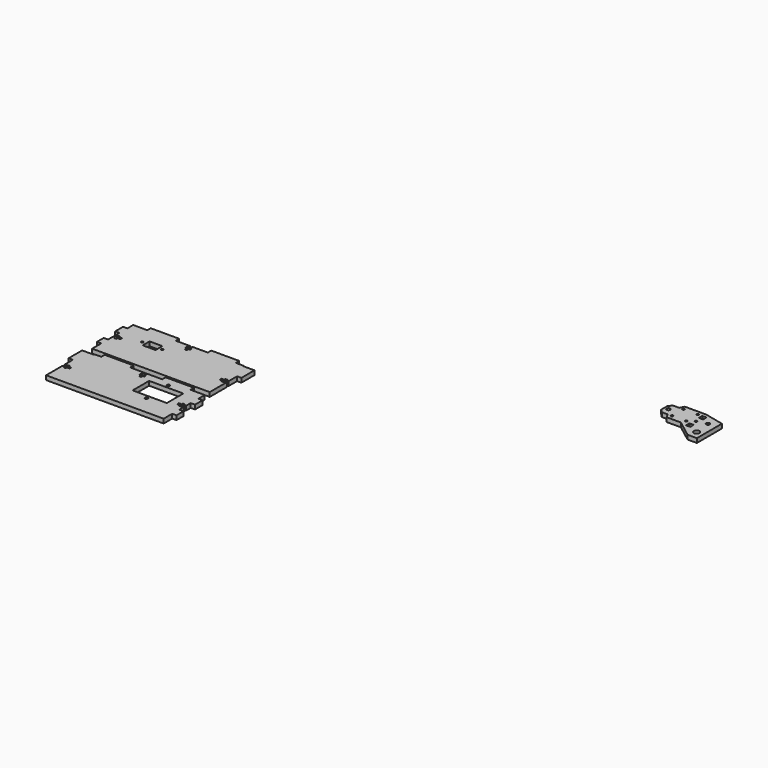
from build123d import *

# Parameters (mm, degrees)
F0_R     = 2
F0_W     = 48
F0_H     = 29
F1_DEPTH = 6
F0_R_2   = 1.5
F0_W_2   = 18
F0_H_2   = 12
F2_DEPTH = 6
F0_R_3   = 4
F0_W_3   = 6
F0_H_3   = 6
F0_R_4   = 2.5
F3_DEPTH = 6


# Not quite as in the source:
# - a feature of the source that left no trace in its solid (it failed there, or was rolled back) is left out


with BuildPart() as f1:
    # F0 (on Top) → F1 (new body)
    with BuildSketch(Plane.XY):
        Polygon((-322.260171175, -178.4142817259), (-362.7690343857, -178.4142817259), (-362.7690343857, -184.4142817259), (-372.3870515823, -184.4142817259), (-372.3870515823, -185.5936968327), (-388.6211997944, -185.5936968327), (-388.6211997944, -209.4142817259), (-382.6211997944, -209.4142817259), (-382.6211997944, -224.8172610998), (-379.3355226517, -224.8172610998), (-379.3355226517, -222.8172610998), (-376.3355226517, -222.8172610998), (-376.3355226517, -224.8172610998), (-372.6211997944, -224.8172610998), (-372.6211997944, -227.8172610998), (-376.2749941349, -227.8172610998), (-376.2749941349, -229.8172610998), (-379.2749941349, -229.8172610998), (-379.2749941349, -227.8172610998), (-382.6211997944, -227.8172610998), (-382.6211997944, -256.4142817259), (-217.6211997944, -256.4142817259), (-217.6211997944, -241.4142817259), (-211.6211997944, -241.4142817259), (-211.6211997944, -228.9265096188), (-217.6211997944, -228.9265096188), (-217.6211997944, -220.2628701925), (-220.4560786486, -220.2628701925), (-220.4560786486, -222.2628701925), (-223.4560786486, -222.2628701925), (-223.4560786486, -220.2628701925), (-227.6211997944, -220.2628701925), (-227.6211997944, -217.2628701925), (-223.4560786486, -217.2628701925), (-223.4560786486, -215.2628701925), (-220.4560786486, -215.2628701925), (-220.4560786486, -217.2628701925), (-217.6211997944, -217.2628701925), (-217.6211997944, -208.9265096188), (-211.6211997944, -208.9265096188), (-211.6211997944, -195.4697817564), (-217.6211997944, -195.4697817564), (-217.6211997944, -184.4142817259), (-237.4467253685, -184.4142817259), (-237.4467253685, -178.4142817259), (-277.260171175, -178.4142817259), (-277.260171175, -184.4142817259), (-298.62987113, -184.4142817259), (-298.62987113, -188.4142817259), (-296.62987113, -188.4142817259), (-296.62987113, -191.4142817259), (-298.62987113, -191.4142817259), (-298.62987113, -194.4142817259), (-301.62987113, -194.4142817259), (-301.62987113, -191.4142817259), (-303.62987113, -191.4142817259), (-303.62987113, -188.4142817259), (-301.62987113, -188.4142817259), (-301.62987113, -184.4142817259), (-322.260171175, -184.4142817259), align=None)
        with Locations((-262.8113031387, -230.070233345)):
            Circle(F0_R, mode=Mode.SUBTRACT)
        with Locations((-262.1210625172, -210.7260148525)):
            Rectangle(F0_W, F0_H, mode=Mode.SUBTRACT)
        with Locations((-262.8113031387, -191.5435940027)):
            Circle(F0_R, mode=Mode.SUBTRACT)
    extrude(amount=F1_DEPTH)


with BuildPart() as f2:
    # F0 (on Top) → F2 (new body)
    with BuildSketch(Plane.XY):
        Polygon((-322.9325413704, -97.594037652), (-362.841963768, -97.594037652), (-362.6211997944, -103.5899748822), (-382.6211997944, -103.5899748822), (-382.6211997944, -113.8526499271), (-388.6211997944, -113.8526499271), (-388.6211997944, -127.7235001326), (-382.6211997944, -127.7235001326), (-382.6211997944, -135.98858428), (-379.6105473042, -135.98858428), (-379.6105473042, -133.98858428), (-376.6105473042, -133.98858428), (-376.6105473042, -135.98858428), (-372.6211997944, -135.98858428), (-372.6211997944, -138.98858428), (-376.6105473042, -138.98858428), (-376.6105473042, -140.98858428), (-379.6105473042, -140.98858428), (-379.6105473042, -138.98858428), (-382.6211997944, -138.98858428), (-382.6211997944, -147.7235001326), (-388.6211997944, -147.7235001326), (-388.6211997944, -159.594037652), (-382.6211997944, -159.594037652), (-382.6211997944, -175.594037652), (-217.6211997944, -175.594037652), (-217.6211997944, -145.6676274538), (-220.7599878311, -145.6676274538), (-220.7599878311, -147.6676274538), (-223.7599878311, -147.6676274538), (-223.7599878311, -145.6676274538), (-227.6211997944, -145.6676274538), (-227.6211997944, -142.6676274538), (-223.7599878311, -142.6676274538), (-223.7599878311, -140.6676274538), (-220.7599878311, -140.6676274538), (-220.7599878311, -142.6676274538), (-217.6211997944, -142.6676274538), (-217.6211997944, -127.594037652), (-211.6211997944, -127.594037652), (-211.6211997944, -104.594037652), (-227.6211997944, -104.594037652), (-227.6211997944, -103.594037652), (-238.6211997944, -103.594037652), (-238.6211997944, -97.594037652), (-277.9325413704, -97.594037652), (-277.9325413704, -103.594037652), (-299.3002493382, -103.594037652), (-299.3002493382, -107.3925257921), (-297.3002493382, -107.3925257921), (-297.3002493382, -110.3925257921), (-299.3002493382, -110.3925257921), (-299.3002493382, -113.594037652), (-302.3002493382, -113.594037652), (-302.3002493382, -110.3925257921), (-304.3002493382, -110.3925257921), (-304.3002493382, -107.3925257921), (-302.3002493382, -107.3925257921), (-302.3002493382, -103.594037652), (-322.9325413704, -103.594037652), align=None)
        with Locations((-349.8402833939, -129.0218681097)):
            Circle(F0_R_2, mode=Mode.SUBTRACT)
        with Locations((-335.2745141983, -128.7626596689)):
            Rectangle(F0_W_2, F0_H_2, mode=Mode.SUBTRACT)
        with Locations((-321.5666413307, -129.0218681097)):
            Circle(F0_R_2, mode=Mode.SUBTRACT)
    extrude(amount=F2_DEPTH)


with BuildPart() as f3:
    # F0 (on Top) → F3 (new body)
    with BuildSketch(Plane.XY):
        Polygon((240.6081428044, 122.7075162329), (210.6081428044, 122.7075162329), (207.3727697134, 116.7111811042), (199.0681737661, 116.7111811042), (194.7087794542, 112.3517867923), (194.7087794542, 101.0705754161), (199.0681737661, 96.7111811042), (207.3727697134, 96.7111811042), (210.6081428044, 90.7075162329), (230.6081428044, 90.7075162329), (254.5574009418, 72.5415870547), (267.5574009418, 72.5415870547), (267.5574009418, 116.5415870547), align=None)
        with Locations((213.1369262934, 97.0565155149)):
            Circle(F0_R_2, mode=Mode.SUBTRACT)
        with Locations((258.2755386829, 83.7381631136)):
            Circle(F0_R_3, mode=Mode.SUBTRACT)
        with Locations((242.166555047, 91.9554172754)):
            Rectangle(F0_W_3, F0_H_3, mode=Mode.SUBTRACT)
        with Locations((233.1369262934, 97.0565155149)):
            Circle(F0_R_2, mode=Mode.SUBTRACT)
        with Locations((200.3271728754, 106.7111811042)):
            Circle(F0_R_4, mode=Mode.SUBTRACT)
        with Locations((213.1369262934, 117.0565155149)):
            Circle(F0_R_2, mode=Mode.SUBTRACT)
        with Locations((241.9558465481, 103.1761914492)):
            Circle(F0_R_2, mode=Mode.SUBTRACT)
        with Locations((255.7267546654, 106.7111811042)):
            Circle(F0_R_4, mode=Mode.SUBTRACT)
        with Locations((242.2060729265, 114.5068718791)):
            Rectangle(F0_W_3, F0_H_3, mode=Mode.SUBTRACT)
        with Locations((233.1369262934, 117.0565155149)):
            Circle(F0_R_2, mode=Mode.SUBTRACT)
    extrude(amount=F3_DEPTH)


solid = Compound([f1.part, f2.part, f3.part])
